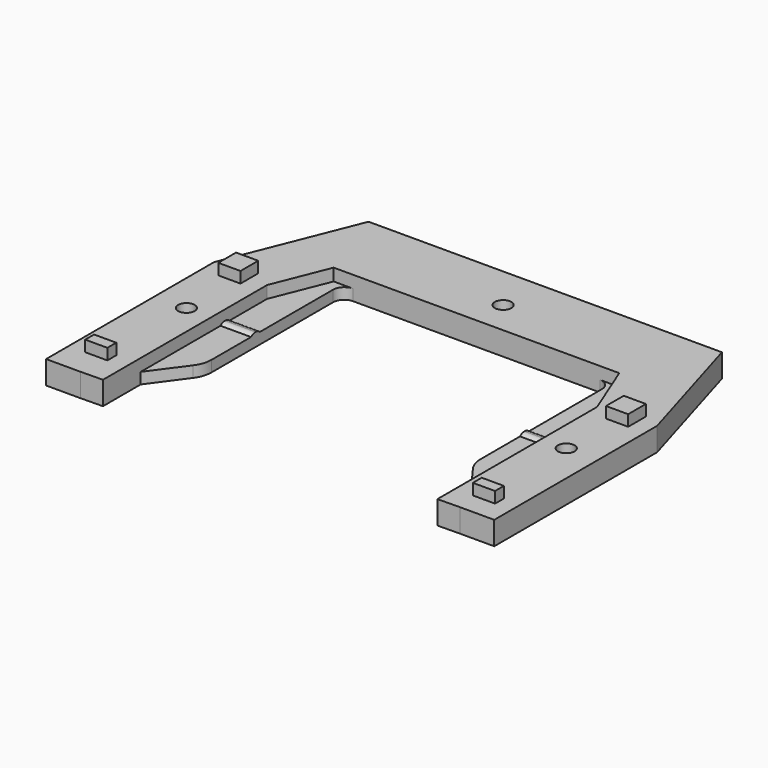
from build123d import *

# Parameters (mm, degrees)
F1_DEPTH      = 2
F2_DEPTH      = 4.2
F3_DEPTH      = 6.2
F4_DEPTH      = 6.2
F5_W          = 4
F5_H          = 2
F5_H_2        = 4
F6_DEPTH      = 2
F7_R          = 2.5
F7_R_2        = 1.5
F8_DEPTH      = 2.5
F9_DEPTH      = 4.5
F10_R         = 5
F12_START     = -1.7
F11_R         = 2.5
F11_R_2       = 1.5
F12_DEPTH     = 5.1
F13_DEPTH     = 4.2
F14_W         = 5.5
F14_H         = 2
F15_DEPTH     = 0.4
F16_T1_DEPTH  = 7.9494897428
F16_T3_DEPTH  = 7.9494897428
F17_S5_R      = 1.5
F17_T6_DEPTH  = 5
F17_S11_R     = 1.5
F17_T12_DEPTH = 5
F17_S17_R     = 1.5
F17_T18_DEPTH = 5


# Not quite as in the source:
# - a fillet or chamfer that OpenCascade refuses, or shapes differently, is made with other operations: its cross-section is extruded or revolved along the edge and cut away or added


with BuildPart() as f1:
    # F0 (on Top) → F1 (new body)
    with BuildSketch(Plane.XY):
        with BuildLine():
            Line((-22, 14.25), (-25.5, 14.25))
            Line((-25.5, 14.25), (-29.5, 4.25))
            Line((-29.5, 4.25), (-29.5, -24.25))
            Line((-29.5, -24.25), (-24, -16.75))
            Line((-24, -16.75), (-24, 12.25))
            ThreePointArc((-24, 12.25), (-23.4142135624, 13.6642135624), (-22, 14.25))
        make_face()
    extrude(amount=F1_DEPTH)



with BuildPart() as f1b:
    # F0 (on Top) → F1, piece 2 (new body)
    with BuildSketch(Plane.XY):
        with BuildLine():
            Line((26, 14.25), (22.5, 14.25))
            ThreePointArc((22.5, 14.25), (23.9142135624, 13.6642135624), (24.5, 12.25))
            Line((24.5, 12.25), (24.5, -16.75))
            Line((24.5, -16.75), (30, -24.25))
            Line((30, -24.25), (30, 4.25))
            Line((30, 4.25), (26, 14.25))
        make_face()
    extrude(amount=F1_DEPTH)


with BuildPart() as f1_1:
    add(f1.part)

    add(f1b.part)  # F2 merges F1b
    # F0 (on Top) → F2 (join)
    with BuildSketch(Plane.XY):
        Polygon((-29.5, 4.25), (-25.5, 14.25), (-22, 14.25), (22.5, 14.25), (26, 14.25), (30, 4.25), (30, -24.25), (30, -31.75), (34, -31.6827731092), (34, 5.0203296143), (27.1081318457, 28.25), (-24.2081318457, 28.25), (-33.5, 5.0203296143), (-33.5, -32.8172268908), (-29.5, -32.75), (-29.5, -24.25), align=None)
    extrude(amount=F2_DEPTH)

    # F3 (add): faces of the model
    f3_faces = [f1_1.faces().sort_by_distance(p)[0] for p in [
        (-33.5, -13.8984486382, 2.1),
        (-28.8540659229, 16.6351648071, 2.1),
    ]]
    extrude(f3_faces, amount=F3_DEPTH, dir=(-1, 0, 0))

    # F4 (add): faces of the model
    f4_faces = [f1_1.faces().sort_by_distance(p)[0] for p in [
        (34, -13.3312217475, 2.1),
        (30.5540659229, 16.6351648071, 2.1),
    ]]
    extrude(f4_faces, amount=F4_DEPTH, dir=(1, 0, 0))

    # F5 (on face) → F6 (join)
    with BuildSketch(Plane.XY.offset(4.2)):
        with Locations((-34.7, -26.75)):
            Rectangle(F5_W, F5_H)
        with Locations((35.2, -26.75)):
            Rectangle(F5_W, F5_H)
        with Locations((35.2, 4.25)):
            Rectangle(F5_W, F5_H_2)
        with Locations((-34.7, 4.25)):
            Rectangle(F5_W, F5_H_2)
    extrude(amount=F6_DEPTH)

    # F7 (on face) → F8 (cut)
    with BuildSketch(Plane(origin=(0, 0, 0), x_dir=(1, 0, 0), z_dir=(0, 0, -1))):
        with Locations((-34, 8.3172268908)):
            Circle(F7_R)
        with Locations((-34, 8.3172268908)):
            Circle(F7_R_2, mode=Mode.SUBTRACT)
        with Locations((34.5, 8.3172268908)):
            Circle(F7_R)
        with Locations((34.5, 8.3172268908)):
            Circle(F7_R_2, mode=Mode.SUBTRACT)
    extrude(amount=-F8_DEPTH, mode=Mode.SUBTRACT)

    # F9 (cut): faces of the model
    f9_faces = [f1_1.faces().sort_by_distance(p)[0] for p in [
        (-34, -8.3172268908, 0),
        (34.5, -8.3172268908, 0),
    ]]
    extrude(f9_faces, amount=-F9_DEPTH, mode=Mode.SUBTRACT)

    # F10
    f10_edges = [f1_1.edges().sort_by_distance(p)[0] for p in [
        (24.5, -16.75, 1),
        (-24, -16.75, 1),
    ]]
    fillet(f10_edges, radius=F10_R)

    # F11 (on face) → F12 (cut)
    with BuildSketch(Plane.XY.offset(4.2).offset(F12_START)):
        with Locations((0.25, 20.25)):
            Circle(F11_R)
        with Locations((0.25, 20.25)):
            Circle(F11_R_2, mode=Mode.SUBTRACT)
    extrude(amount=-F12_DEPTH, mode=Mode.SUBTRACT)

    # F11 (on face) → F13 (cut)
    with BuildSketch(Plane.XY.offset(4.2)):
        with Locations((0.25, 20.25)):
            Circle(F11_R_2)
    extrude(amount=-F13_DEPTH, mode=Mode.SUBTRACT)

    # F14 (on face) → F15 (join)
    with BuildSketch(Plane.XY.offset(2)):
        with Locations((27.25, -5.25)):
            Rectangle(F14_W, F14_H)
        with Locations((-26.75, -5.25)):
            Rectangle(F14_W, F14_H)
    extrude(amount=F15_DEPTH)

    # F16: fillet of radius 1.4 on 4 edges, made by hand

    # F16_s2 → F16_t1 (cut)
    with BuildSketch(Plane.YZ.offset(-29.5)):
        with BuildLine():
            ThreePointArc((-6.25, 2), (-5.7993543651, 2.2961481397), (-5.2702041029, 2.4))
            Line((-5.2702041029, 2.4), (-6.25, 2.4))
            Line((-6.25, 2.4), (-6.25, 2))
        make_face()
        with BuildLine():
            ThreePointArc((-5.2297958971, 2.4), (-4.7006456349, 2.2961481397), (-4.25, 2))
            Line((-4.25, 2), (-4.25, 2.4))
            Line((-4.25, 2.4), (-5.2297958971, 2.4))
        make_face()
    extrude(amount=F16_T1_DEPTH, mode=Mode.SUBTRACT)

    # F16_s4 → F16_t3 (cut)
    with BuildSketch(Plane.YZ.offset(22.0505102572)):
        with BuildLine():
            ThreePointArc((-4.25, 2), (-4.7006456349, 2.2961481397), (-5.2297958971, 2.4))
            Line((-5.2297958971, 2.4), (-4.25, 2.4))
            Line((-4.25, 2.4), (-4.25, 2))
        make_face()
        with BuildLine():
            ThreePointArc((-6.25, 2), (-5.7993543651, 2.2961481397), (-5.2702041029, 2.4))
            Line((-5.2702041029, 2.4), (-6.25, 2.4))
            Line((-6.25, 2.4), (-6.25, 2))
        make_face()
    extrude(amount=F16_T3_DEPTH, mode=Mode.SUBTRACT)

    # F17: chamfer of 1.2 on 3 edges, made by hand


with BuildPart() as f17_tool2:
    # F17_s3 → F17_t4 (revolve)
    with BuildSketch(Plane.XZ.offset(8.3172268908)):
        Polygon((-31.5, 1.3), (-32.7, 2.5), (-31.5, 2.5), align=None)
    revolve(axis=Axis((-34, -8.3172268908, 2.5), (0, 0, -1)))

    # F17_s5 → F17_t6 (cut, symmetric)
    with BuildSketch(Plane.XY.offset(1.9)):
        with Locations((-34, -8.3172268908)):
            Circle(F17_S5_R)
    extrude(amount=F17_T6_DEPTH, both=True, mode=Mode.SUBTRACT)


with BuildPart() as f1_2:
    add(f1_1.part)

    # F17_t1: union F17_tool2
    add(f17_tool2.part)


with BuildPart() as f17_tool8:
    # F17_s9 → F17_t10 (revolve)
    with BuildSketch(Plane.XZ.offset(8.3172268908)):
        Polygon((37, 1.3), (35.8, 2.5), (37, 2.5), align=None)
    revolve(axis=Axis((34.5, -8.3172268908, 2.5), (0, 0, -1)))

    # F17_s11 → F17_t12 (cut, symmetric)
    with BuildSketch(Plane.XY.offset(1.9)):
        with Locations((34.5, -8.3172268908)):
            Circle(F17_S11_R)
    extrude(amount=F17_T12_DEPTH, both=True, mode=Mode.SUBTRACT)


with BuildPart() as f1_3:
    add(f1_2.part)

    # F17_t7: union F17_tool8
    add(f17_tool8.part)


with BuildPart() as f17_tool14:
    # F17_s15 → F17_t16 (revolve)
    with BuildSketch(Plane.XZ.offset(-20.25)):
        Polygon((2.75, 1.3), (1.55, 2.5), (2.75, 2.5), align=None)
    revolve(axis=Axis((0.25, 20.25, 2.5), (0, 0, 1)))

    # F17_s17 → F17_t18 (cut, symmetric)
    with BuildSketch(Plane.XY.offset(1.9)):
        with Locations((0.25, 20.25)):
            Circle(F17_S17_R)
    extrude(amount=F17_T18_DEPTH, both=True, mode=Mode.SUBTRACT)


with BuildPart() as f1_4:
    add(f1_3.part)

    # F17_t13: union F17_tool14
    add(f17_tool14.part)


solid = f1_4.part
